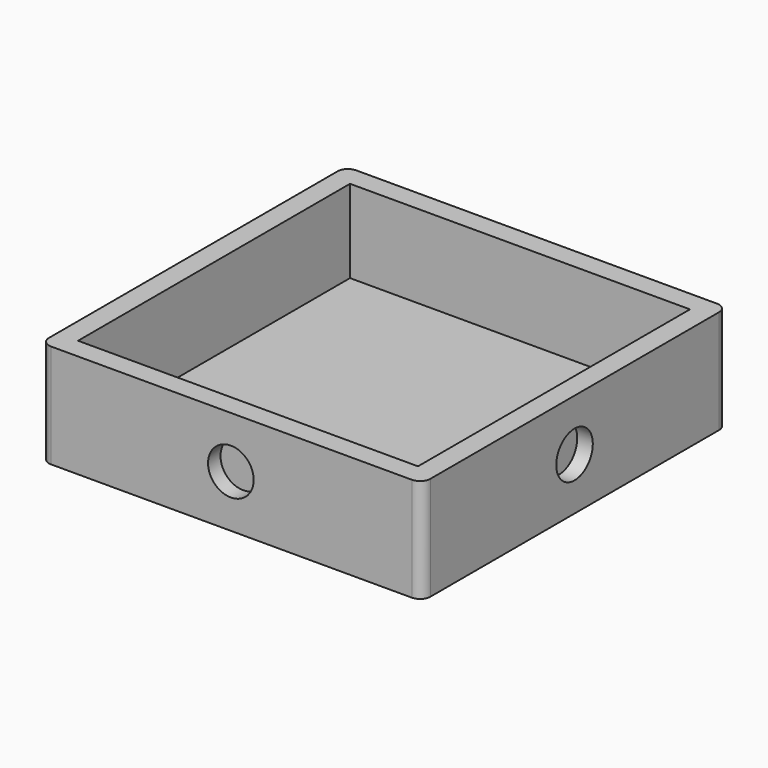
from build123d import *

# Parameters (mm, degrees)
F0_W        = 65.5
F0_H        = 65.5
F1_DEPTH    = 16
F2_T        = 4
F3_T1_DEPTH = 30
F4_R        = 4.4
F8_DEPTH    = 3
F9_DEPTH    = 3
F5_R        = 4.4
F10_DEPTH   = 3
F6_R        = 4.4
F11_DEPTH   = 3
F7_R        = 4.4
F12_DEPTH   = 3


# Not quite as in the source:
# - a fillet or chamfer that OpenCascade refuses, or shapes differently, is made with other operations: its cross-section is extruded or revolved along the edge and cut away or added


with BuildPart() as f1:
    # F0 (on Top) → F1 (new body)
    with BuildSketch(Plane.XY):
        with Locations((4.3041806072, -3.8802318871)):
            Rectangle(F0_W, F0_H)
    extrude(amount=F1_DEPTH)

    # F2
    f2_openings = [f1.faces().sort_by_distance(p)[0] for p in [
        (4.304181, -3.880232, 16),
    ]]
    offset(amount=F2_T, openings=f2_openings, kind=Kind.INTERSECTION)

    # F3: fillet of radius 2 on 4 edges, made by hand

    # F3_s2 → F3_t1 (cut)
    with BuildSketch(Plane.XY.offset(-9)):
        with BuildLine():
            ThreePointArc((41.0541806072, -38.6302318871), (40.4683941696, -40.0444454495), (39.0541806072, -40.6302318871))
            Line((39.0541806072, -40.6302318871), (41.0541806072, -40.6302318871))
            Line((41.0541806072, -40.6302318871), (41.0541806072, -38.6302318871))
        make_face()
        with BuildLine():
            ThreePointArc((41.0541806072, 30.8697681129), (40.4683941696, 32.2839816753), (39.0541806072, 32.8697681129))
            Line((39.0541806072, 32.8697681129), (41.0541806072, 32.8697681129))
            Line((41.0541806072, 32.8697681129), (41.0541806072, 30.8697681129))
        make_face()
        with BuildLine():
            ThreePointArc((-30.4458193928, 32.8697681129), (-31.8600329552, 32.2839816753), (-32.4458193928, 30.8697681129))
            Line((-32.4458193928, 30.8697681129), (-32.4458193928, 32.8697681129))
            Line((-32.4458193928, 32.8697681129), (-30.4458193928, 32.8697681129))
        make_face()
        with BuildLine():
            ThreePointArc((-32.4458193928, -38.6302318871), (-31.8600329552, -40.0444454495), (-30.4458193928, -40.6302318871))
            Line((-30.4458193928, -40.6302318871), (-32.4458193928, -40.6302318871))
            Line((-32.4458193928, -40.6302318871), (-32.4458193928, -38.6302318871))
        make_face()
    extrude(amount=F3_T1_DEPTH, mode=Mode.SUBTRACT)

    # F4 (on face) → F8 (join)
    with BuildSketch(Plane(origin=(-32.4458193928, 0, 0), x_dir=(0, -1, 0), z_dir=(-1, 0, 0))):
        with Locations((3.8802318871, 6)):
            Circle(F4_R)
    extrude(amount=-F8_DEPTH)

    # F4 (on face) → F9 (cut)
    with BuildSketch(Plane(origin=(-32.4458193928, 0, 0), x_dir=(0, -1, 0), z_dir=(-1, 0, 0))):
        with Locations((3.8802318871, 6)):
            Circle(F4_R)
    extrude(amount=-F9_DEPTH, mode=Mode.SUBTRACT)

    # F5 (on face) → F10 (cut)
    with BuildSketch(Plane.XZ.offset(40.6302318871)):
        with Locations((4.2000180173, 6.0547004089)):
            Circle(F5_R)
    extrude(amount=-F10_DEPTH, mode=Mode.SUBTRACT)

    # F6 (on face) → F11 (cut)
    with BuildSketch(Plane.YZ.offset(41.0541806072)):
        with Locations((-3.9293510383, 6.0207889489)):
            Circle(F6_R)
    extrude(amount=-F11_DEPTH, mode=Mode.SUBTRACT)

    # F7 (on face) → F12 (cut)
    with BuildSketch(Plane(origin=(0, 32.8697681129, 0), x_dir=(-1, 0, 0), z_dir=(0, 1, 0))):
        with Locations((-4.345219037, 6.0662772571)):
            Circle(F7_R)
    extrude(amount=-F12_DEPTH, mode=Mode.SUBTRACT)


solid = f1.part
